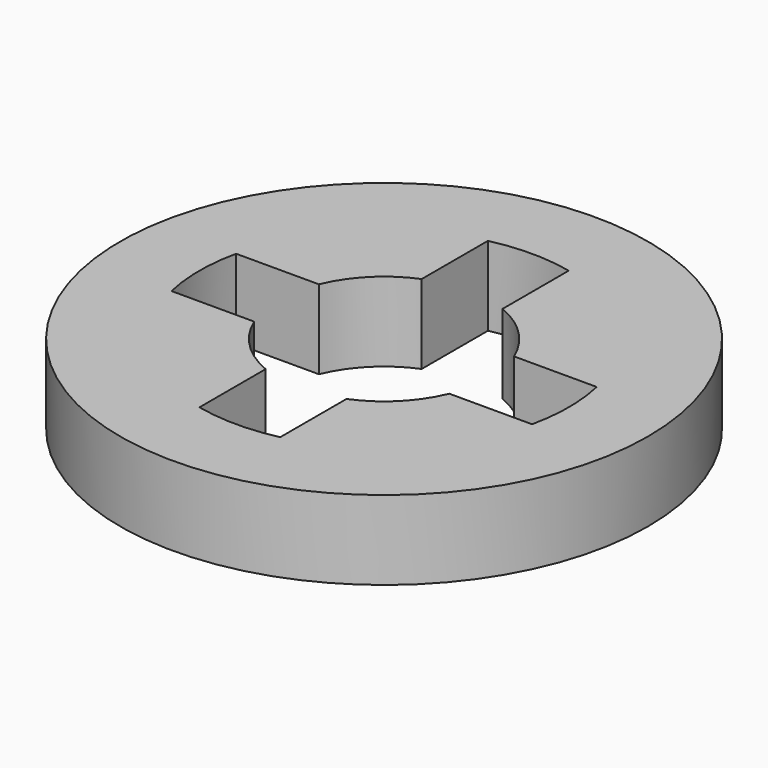
from build123d import *

# Parameters (mm, degrees)
F0_R            = 33.335
F1_DEPTH        = 10
F2_R            = 13.335
F3_DEPTH        = 10
F5_DEPTH        = 10
F5_COPIES_COUNT = 4


# Not quite as in the source:
# - a pattern or mirror of a feature is missing from the dataset's text; its kind, count and spacing are read off the source's solid


with BuildPart() as f1:
    # F0 (on Top) → F1 (new body)
    with BuildSketch(Plane.XY):
        Circle(F0_R)
    extrude(amount=F1_DEPTH)

    # F2 (on face) → F3 (cut, through all)
    with BuildSketch(Plane.XY.offset(10)):
        Circle(F2_R)
    extrude(amount=-F3_DEPTH, mode=Mode.SUBTRACT)

    # F4 (on Top) → F5 (cut, through all)
    with BuildSketch(Plane.XY):
        with BuildLine():
            Line((22.7701726623, 5.1030835706), (12.319933566, 5.1030835706))
            ThreePointArc((12.319933566, 5.1030835706), (13.335, 0), (12.319933566, -5.1030835706))
            Line((12.319933566, -5.1030835706), (22.7701726623, -5.1030835706))
            ThreePointArc((22.7701726623, -5.1030835706), (23.335, 0), (22.7701726623, 5.1030835706))
        make_face()
    f5 = extrude(amount=F5_DEPTH, mode=Mode.SUBTRACT)

    # F5_copies: F5 ×4 about axis
    f5_copies_axis = Axis((0, 0, 0), (0, 0, 1))
    for i in range(1, F5_COPIES_COUNT):
        add(f5.rotate(f5_copies_axis, i * 360 / F5_COPIES_COUNT), mode=Mode.SUBTRACT)


solid = f1.part
